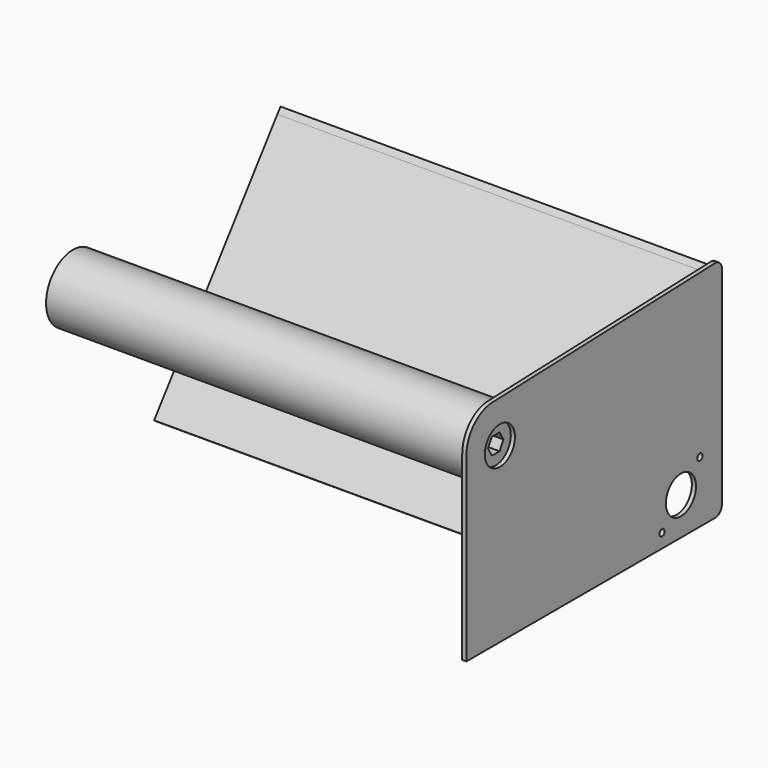
from build123d import *

# Parameters (mm, degrees)
F0_R     = 2.4892
F0_R_2   = 14.2875
F1_DEPTH = 3.175
F2_DEPTH = 320.675
F3_DEPTH = 327.025
F5_R     = 6.35


# Not quite as in the source:
# - the program builds the solid bodies; features that only make, move or delete a surface that nothing else refers to are left out


with BuildPart() as f1:
    # F0 (on Right) → F1 (new body)
    with BuildSketch(Plane.YZ):
        with BuildLine():
            ThreePointArc((4.5600132785, -24.9873223635), (-21.7962589324, 13.0415910284), (24.1745661853, 7.7942510707))
            Line((24.1745661853, 7.7942510707), (134.6951456058, -58.3347209468))
            Line((134.6951456058, -58.3347209468), (201.7698075546, 31.75))
            Line((201.7698075546, 31.75), (-6.35, 31.75))
            ThreePointArc((-6.35, 31.75), (-24.3105122421, 24.3105122421), (-31.75, 6.35))
            Line((-31.75, 6.35), (-31.75, -131.2644877579))
            Line((-31.75, -131.2644877579), (210.4560597146, -131.2644877579))
            Line((210.4560597146, -131.2644877579), (210.4560597146, 31.75))
            Line((210.4560597146, 31.75), (205.7282433529, 31.75))
            Line((205.7282433529, 31.75), (137.4335839182, -59.9732403202))
            Line((137.4335839182, -59.9732403202), (181.4310192869, -86.2987010407))
            ThreePointArc((181.4310192869, -86.2987010407), (188.0145295507, -112.4967642112), (161.8164663801, -119.080274475))
            Line((161.8164663801, -119.080274475), (114.5027408261, -90.7705420286))
            Line((114.5027408261, -90.7705420286), (87.5272601843, -127))
            Line((87.5272601843, -127), (84.9806418952, -125.1038564691))
            Line((84.9806418952, -125.1038564691), (111.7643025136, -89.1320226553))
            Line((111.7643025136, -89.1320226553), (4.5600132785, -24.9873223635))
        make_face()
        with Locations((153.6632305914, -120.65)):
            Circle(F0_R, mode=Mode.SUBTRACT)
        with Locations((189.5842550757, -84.7289755157)):
            Circle(F0_R, mode=Mode.SUBTRACT)
        with BuildLine():
            ThreePointArc((24.1745661853, 7.7942510707), (25.0917713714, 3.9449980288), (25.4, 0))
            ThreePointArc((25.4, 0), (19.5062084639, -16.2686149184), (4.5600132785, -24.9873223635))
            Line((4.5600132785, -24.9873223635), (111.7643025136, -89.1320226553))
            Line((111.7643025136, -89.1320226553), (134.6951456058, -58.3347209468))
            Line((134.6951456058, -58.3347209468), (24.1745661853, 7.7942510707))
        make_face()
        with BuildLine():
            Line((9.8072764534, 16.3907867171), (24.1745661853, 7.7942510707))
            ThreePointArc((24.1745661853, 7.7942510707), (-21.7962589324, 13.0415910284), (4.5600132785, -24.9873223635))
            Line((4.5600132785, -24.9873223635), (-9.8072764534, -16.3907867171))
            ThreePointArc((-9.8072764534, -16.3907867171), (-16.3907867171, 9.8072764534), (9.8072764534, 16.3907867171))
        make_face()
        with BuildLine():
            ThreePointArc((4.5600132785, -24.9873223635), (19.5062084639, -16.2686149184), (25.4, 0))
            ThreePointArc((25.4, 0), (25.0917713714, 3.9449980288), (24.1745661853, 7.7942510707))
            Line((24.1745661853, 7.7942510707), (9.8072764534, 16.3907867171))
            ThreePointArc((9.8072764534, 16.3907867171), (-16.3907867171, 9.8072764534), (-9.8072764534, -16.3907867171))
            Line((-9.8072764534, -16.3907867171), (4.5600132785, -24.9873223635))
        make_face()
        Circle(F0_R_2, mode=Mode.SUBTRACT)
        Polygon((114.5027408261, -90.7705420286), (111.7643025136, -89.1320226553), (84.9806418952, -125.1038564691), (87.5272601843, -127), align=None)
        Polygon((137.4335839182, -59.9732403202), (134.6951456058, -58.3347209468), (111.7643025136, -89.1320226553), (114.5027408261, -90.7705420286), align=None)
        Polygon((201.7698075546, 31.75), (134.6951456058, -58.3347209468), (137.4335839182, -59.9732403202), (205.7282433529, 31.75), align=None)
        Polygon((204.7344414256, 35.731655773), (201.7698075546, 31.75), (205.7282433529, 31.75), (207.2810597146, 33.8355122421), align=None)
        with BuildLine():
            Line((181.4310192869, -86.2987010407), (137.4335839182, -59.9732403202))
            Line((137.4335839182, -59.9732403202), (114.5027408261, -90.7705420286))
            Line((114.5027408261, -90.7705420286), (161.8164663801, -119.080274475))
            ThreePointArc((161.8164663801, -119.080274475), (188.0145295507, -112.4967642112), (181.4310192869, -86.2987010407))
        make_face()
        with Locations((171.6237428335, -102.6894877579)):
            Circle(F0_R_2, mode=Mode.SUBTRACT)
        Polygon((-6.35, 31.75), (201.7698075546, 31.75), (204.7344414256, 35.731655773), (207.2810597146, 33.8355122421), (205.7282433529, 31.75), (210.4560597146, 31.75), (210.4560597146, 39.1025175512), align=None)
    extrude(amount=F1_DEPTH)

    # F5
    f5_edges = [f1.edges().sort_by_distance(p)[0] for p in [
        (1.5875, -6.35, 31.75),
        (1.5875, 210.45606, -131.264488),
        (1.5875, 210.45606, 39.102518),
    ]]
    fillet(f5_edges, radius=F5_R)


with BuildPart() as f2:
    # F0 (on Right) → F2 (new body)
    with BuildSketch(Plane.YZ):
        with BuildLine():
            ThreePointArc((4.5600132785, -24.9873223635), (19.5062084639, -16.2686149184), (25.4, 0))
            ThreePointArc((25.4, 0), (25.0917713714, 3.9449980288), (24.1745661853, 7.7942510707))
            Line((24.1745661853, 7.7942510707), (9.8072764534, 16.3907867171))
            ThreePointArc((9.8072764534, 16.3907867171), (-16.3907867171, 9.8072764534), (-9.8072764534, -16.3907867171))
            Line((-9.8072764534, -16.3907867171), (4.5600132785, -24.9873223635))
        make_face()
        Circle(F0_R_2, mode=Mode.SUBTRACT)
        Circle(F0_R_2)
        Polygon((-7.3323484187, 0), (-3.6661742094, 6.35), (3.6661742094, 6.35), (7.3323484187, 0), (3.6661742094, -6.35), (-3.6661742094, -6.35), align=None, mode=Mode.SUBTRACT)
        with BuildLine():
            Line((9.8072764534, 16.3907867171), (24.1745661853, 7.7942510707))
            ThreePointArc((24.1745661853, 7.7942510707), (-21.7962589324, 13.0415910284), (4.5600132785, -24.9873223635))
            Line((4.5600132785, -24.9873223635), (-9.8072764534, -16.3907867171))
            ThreePointArc((-9.8072764534, -16.3907867171), (-16.3907867171, 9.8072764534), (9.8072764534, 16.3907867171))
        make_face()
    extrude(amount=-F2_DEPTH)


with BuildPart() as f3:
    # F0 (on Right) → F3 (new body)
    with BuildSketch(Plane.YZ):
        Polygon((114.5027408261, -90.7705420286), (111.7643025136, -89.1320226553), (84.9806418952, -125.1038564691), (87.5272601843, -127), align=None)
        Polygon((137.4335839182, -59.9732403202), (134.6951456058, -58.3347209468), (111.7643025136, -89.1320226553), (114.5027408261, -90.7705420286), align=None)
        Polygon((201.7698075546, 31.75), (134.6951456058, -58.3347209468), (137.4335839182, -59.9732403202), (205.7282433529, 31.75), align=None)
        Polygon((204.7344414256, 35.731655773), (201.7698075546, 31.75), (205.7282433529, 31.75), (207.2810597146, 33.8355122421), align=None)
    extrude(amount=-F3_DEPTH)


solid = Compound([f1.part, f2.part, f3.part])
